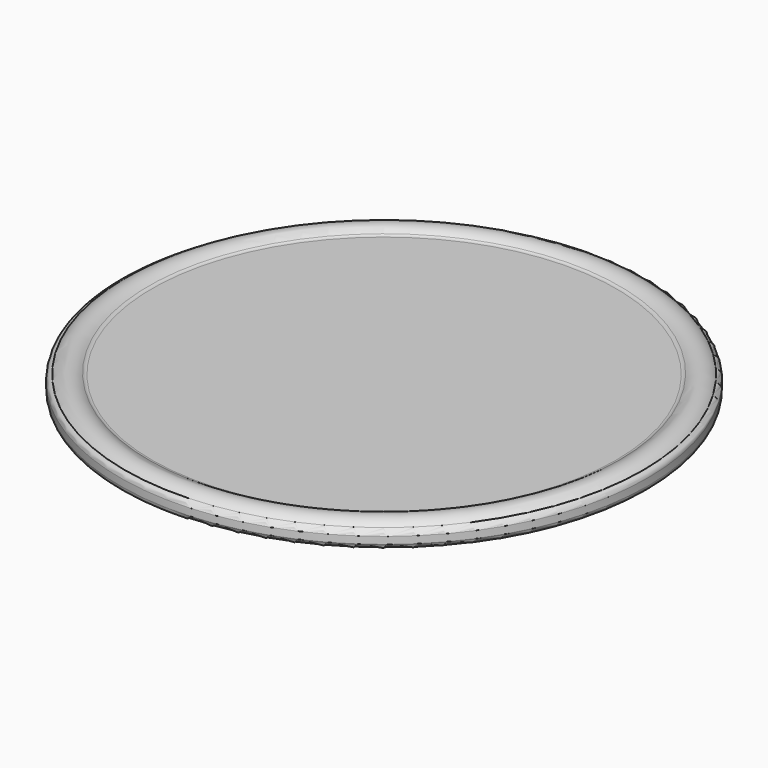
from build123d import *

# Parameters (mm, degrees)
F0_R     = 150
F1_DEPTH = 10


# Not quite as in the source:
# - a fillet or chamfer that OpenCascade refuses, or shapes differently, is made with other operations: its cross-section is extruded or revolved along the edge and cut away or added


with BuildPart() as f1:
    # F0 (on Top) → F1 (new body)
    with BuildSketch(Plane.XY):
        Circle(F0_R)
    extrude(amount=F1_DEPTH)

    # F2 (on Front) → F3 (revolve)
    with BuildSketch(Plane.XZ):
        with BuildLine():
            Line((130.4040820577, 5), (150, 5))
            ThreePointArc((150, 5), (140.2020410289, 13), (130.4040820577, 5))
        make_face()
    revolve(axis=Axis((0, 0, 19.3104613572), (0, 0, 1)))

    # F4: fillet of radius 3 on 4 edges, made by hand

    # F4_s1 → F4_t2 (revolve)
    with BuildSketch(Plane.XZ):
        with BuildLine():
            ThreePointArc((133.8123303651, 10.6923076923), (132.9144664967, 10.1783801706), (131.8954171659, 10))
            Line((131.8954171659, 10), (133.0606126003, 10))
            ThreePointArc((133.0606126003, 10), (133.4276219564, 10.3557627905), (133.8123303651, 10.6923076923))
        make_face()
    revolve(axis=Axis((0, 0, 10), (0, 0, 1)))

    # F4_s3 → F4_t4 (revolve, cut)
    with BuildSketch(Plane.XZ):
        with BuildLine():
            ThreePointArc((150, 3), (149.1213203436, 0.8786796564), (147, 0))
            Line((147, 0), (150, 0))
            Line((150, 0), (150, 3))
        make_face()
    revolve(axis=Axis((0, 0, 0), (0, 0, 1)), mode=Mode.SUBTRACT)

    # F4_s5 → F4_t6 (revolve, cut)
    with BuildSketch(Plane.XZ):
        with BuildLine():
            ThreePointArc((150, 7.0197267354), (149.2394651563, 9.01592207), (147.3434694574, 10))
            Line((147.3434694574, 10), (150, 10))
            Line((150, 10), (150, 7.0197267354))
        make_face()
    revolve(axis=Axis((0, 0, 10), (0, 0, 1)), mode=Mode.SUBTRACT)


solid = f1.part
